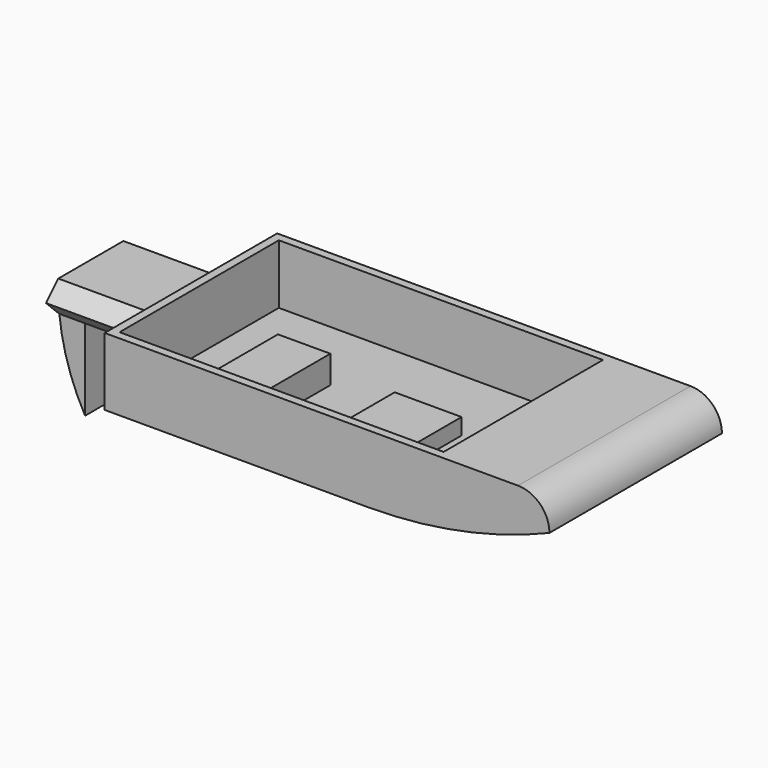
from build123d import *

# Parameters (mm, degrees)
F0_W         = 104.6384423971
F0_H         = 66.2396028638
F1_DEPTH     = 20.828
F2_T         = -2.54
F3_W         = 66.2396028638
F3_H         = 20.828
F4_DEPTH     = 32
F5_R         = 9.6568542495
F6_T1_DEPTH  = 345.145917421
F7_W         = 20.5460339785
F7_H         = 23.8647740334
F8_DEPTH     = 5
F9_W         = 16.0981267691
F9_H         = 24.2720488459
F10_DEPTH    = 8.5
F11_W        = 29.9789980054
F11_H        = 9.4382646494
F12_DEPTH    = 33.9
F13_T1_DEPTH = 46.7584149398
F14_W        = 8.2249975145
F14_H        = 19.9789980054
F15_DEPTH    = 25
F16_T1_DEPTH = 176.8838374013


# Not quite as in the source:
# - a fillet or chamfer that OpenCascade refuses, or shapes differently, is made with other operations: its cross-section is extruded or revolved along the edge and cut away or added


with BuildPart() as f1:
    # F0 (on Top) → F1 (new body)
    with BuildSketch(Plane.XY):
        with Locations((52.3192211986, -33.1198014319)):
            Rectangle(F0_W, F0_H)
    extrude(amount=F1_DEPTH)

    # F2
    f2_openings = [f1.faces().sort_by_distance(p)[0] for p in [
        (52.319221, -33.119801, 20.828),
    ]]
    offset(amount=F2_T, openings=f2_openings)

    # F3 (on face) → F4 (join)
    with BuildSketch(Plane.YZ.offset(104.6384423971)):
        with Locations((-33.1198014319, 10.414)):
            Rectangle(F3_W, F3_H)
    extrude(amount=F4_DEPTH)

    # F5
    f5_edges = [f1.edges().sort_by_distance(p)[0] for p in [
        (136.638442, -33.119801, 20.828),
    ]]
    fillet(f5_edges, radius=F5_R)

    # F6: fillet of radius 144.8528137424 on 1 edges, made by hand

    # F6_s2 → F6_t1 (cut)
    with BuildSketch(Plane.XZ.offset(-139.4531572786)):
        with BuildLine():
            ThreePointArc((136.6384423971, 11.1711457505), (109.301615626, 2.8202410636), (80.8571794857, 0))
            Line((80.8571794857, 0), (80.8571794857, -2.8970562748))
            Line((80.8571794857, -2.8970562748), (136.6384423971, -2.8970562748))
            Line((136.6384423971, -2.8970562748), (139.535498672, 0))
            ThreePointArc((139.535498672, 0), (139.535498672, 5.5855728753), (137.7540676553, 8.4975123907))
            Line((137.7540676553, 8.4975123907), (136.6384423971, 11.1711457505))
        make_face()
    extrude(amount=F6_T1_DEPTH, mode=Mode.SUBTRACT)

    # F7 (on face) → F8 (join)
    with BuildSketch(Plane.XY.offset(2.54)):
        with Locations((67.9204389453, -38.8555312529)):
            Rectangle(F7_W, F7_H)
    extrude(amount=F8_DEPTH)

    # F9 (on face) → F10 (join)
    with BuildSketch(Plane.XY.offset(2.54)):
        with Locations((29.2158611119, -38.2969966158)):
            Rectangle(F9_W, F9_H)
    extrude(amount=F10_DEPTH)

    # F11 (on face) → F12 (join)
    with BuildSketch(Plane(origin=(0, 0, 0), x_dir=(0, -1, 0), z_dir=(-1, 0, 0))):
        with Locations((31.6863805056, 9.8113485146)):
            Rectangle(F11_W, F11_H)
    extrude(amount=F12_DEPTH)

    # F13: chamfer of 5 on 3 edges, made by hand

    # F13_s2 → F13_t1 (cut)
    with BuildSketch(Plane.YZ.offset(-46.7584149398)):
        Polygon((-46.6758795083, 10.09221619), (-41.6758795083, 5.09221619), (-46.6758795083, 5.09221619), align=None)
        Polygon((-21.6968815029, 5.09221619), (-16.6968815029, 10.09221619), (-16.6968815029, 5.09221619), align=None)
        Polygon((-46.6758795083, 9.5304808393), (-41.6758795083, 14.5304808393), (-46.6758795083, 14.5304808393), align=None)
    extrude(amount=F13_T1_DEPTH, mode=Mode.SUBTRACT)

    # F14 (on face) → F15 (join)
    with BuildSketch(Plane(origin=(0, 0, 5.09221619), x_dir=(1, 0, 0), z_dir=(0, 0, -1))):
        with Locations((-29.7875012428, 31.6863805056)):
            Rectangle(F14_W, F14_H)
    extrude(amount=F15_DEPTH)

    # F16: fillet of radius 63.9766594029 on 1 edges, made by hand

    # F16_s2 → F16_t1 (cut)
    with BuildSketch(Plane.XZ.offset(-56.7555381951)):
        with BuildLine():
            ThreePointArc((-33.9, 11.4731840691), (-31.8095992986, -4.7472947243), (-25.6750024855, -19.90778381))
            Line((-25.6750024855, -19.90778381), (-33.9, -19.90778381))
            Line((-33.9, -19.90778381), (-33.9, 11.4731840691))
        make_face()
    extrude(amount=F16_T1_DEPTH, mode=Mode.SUBTRACT)


solid = f1.part
